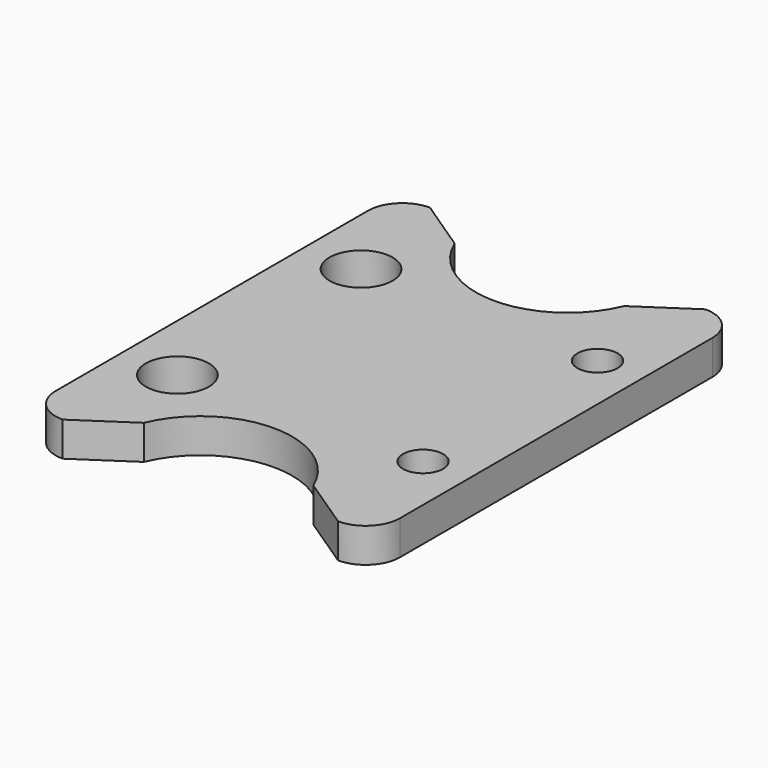
from build123d import *

# Parameters (mm, degrees)
F5_W        = 30
F5_H        = 40
F6_DEPTH    = 3
F8_D        = 5.5
F9_D        = 3.5
F1_DEPTH    = 25
F2_R        = 3
F3_T1_DEPTH = 23.839434056
F4_T1_DEPTH = 23.839434056


# Not quite as in the source:
# - a fillet or chamfer that OpenCascade refuses, or shapes differently, is made with other operations: its cross-section is extruded or revolved along the edge and cut away or added


with BuildPart() as f6:
    # F5 (on Top) → F6 (new body)
    with BuildSketch(Plane.XY):
        Rectangle(F5_W, F5_H)
    extrude(amount=F6_DEPTH)

    # F8 (through all)
    with Locations(Plane.XY.offset(3)):
        with Locations((-10, 10), (-10, -10)):
            Hole(F8_D / 2)

    # F9 (through all)
    with Locations(Plane.XY.offset(3)):
        with Locations((11, 9.5), (11, -9.5)):
            Hole(F9_D / 2)

    # F0 (on face) → F1 (cut)
    with BuildSketch(Plane.XY.offset(3)):
        with BuildLine():
            Line((-8, -20), (8, -20))
            ThreePointArc((8, -20), (0, -12), (-8, -20))
        make_face()
        with BuildLine():
            ThreePointArc((-8, 20), (0, 12), (8, 20))
            Line((8, 20), (-8, 20))
        make_face()
    extrude(amount=-F1_DEPTH, mode=Mode.SUBTRACT)

    # F2
    f2_edges = [f6.edges().sort_by_distance(p)[0] for p in [
        (15, -20, 1.5),
        (-15, -20, 1.5),
        (15, 20, 1.5),
        (-15, 20, 1.5),
    ]]
    fillet(f2_edges, radius=F2_R)

    # F3: chamfer of 5 on 2 edges, made by hand

    # F3_s2 → F3_t1 (cut)
    with BuildSketch(Plane.XY.offset(-10.419717028)):
        with BuildLine():
            Line((-12, 20), (-7.3846153846, 16.9230769231))
            ThreePointArc((-7.3846153846, 16.9230769231), (-7.8300507328, 18.3597849159), (-8, 20))
            Line((-8, 20), (-12, 20))
        make_face()
        with BuildLine():
            Line((7.3846153846, 16.9230769231), (12, 20))
            Line((12, 20), (8, 20))
            ThreePointArc((8, 20), (7.8300507328, 18.3597849159), (7.3846153846, 16.9230769231))
        make_face()
    extrude(amount=F3_T1_DEPTH, mode=Mode.SUBTRACT)

    # F4: chamfer of 5 on 2 edges, made by hand

    # F4_s2 → F4_t1 (cut)
    with BuildSketch(Plane.XY.offset(-10.419717028)):
        with BuildLine():
            Line((7.3846153846, -16.9230769231), (12, -20))
            Line((12, -20), (8, -20))
            ThreePointArc((8, -20), (7.8300507328, -18.3597849159), (7.3846153846, -16.9230769231))
        make_face()
        with BuildLine():
            Line((-12, -20), (-7.3846153846, -16.9230769231))
            ThreePointArc((-7.3846153846, -16.9230769231), (-7.8300507328, -18.3597849159), (-8, -20))
            Line((-8, -20), (-12, -20))
        make_face()
    extrude(amount=F4_T1_DEPTH, mode=Mode.SUBTRACT)


solid = f6.part
